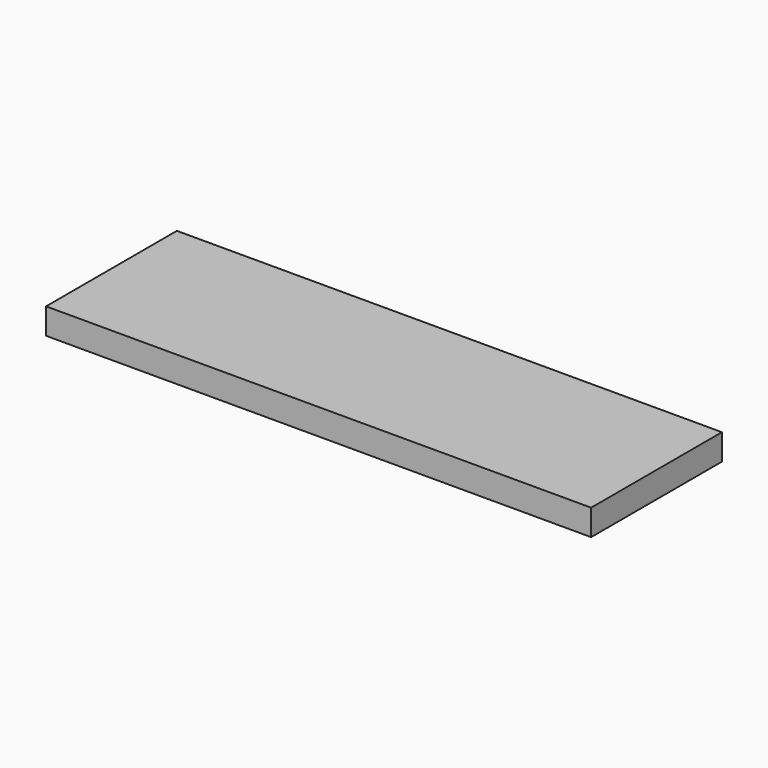
from build123d import *

# Parameters (mm, degrees)
F0_W     = 33.3375
F0_H     = 10
F1_DEPTH = 1.5875


# Not quite as in the source:
# - a length typed as a fraction of an inch, garbled in the dataset ("3 / 203.2 mm" for 3/8 in), is restored


with BuildPart() as f1:
    # F0 (on Top) → F1 (new body)
    with BuildSketch(Plane.XY):
        Rectangle(F0_W, F0_H)
    extrude(amount=F1_DEPTH)


solid = f1.part
